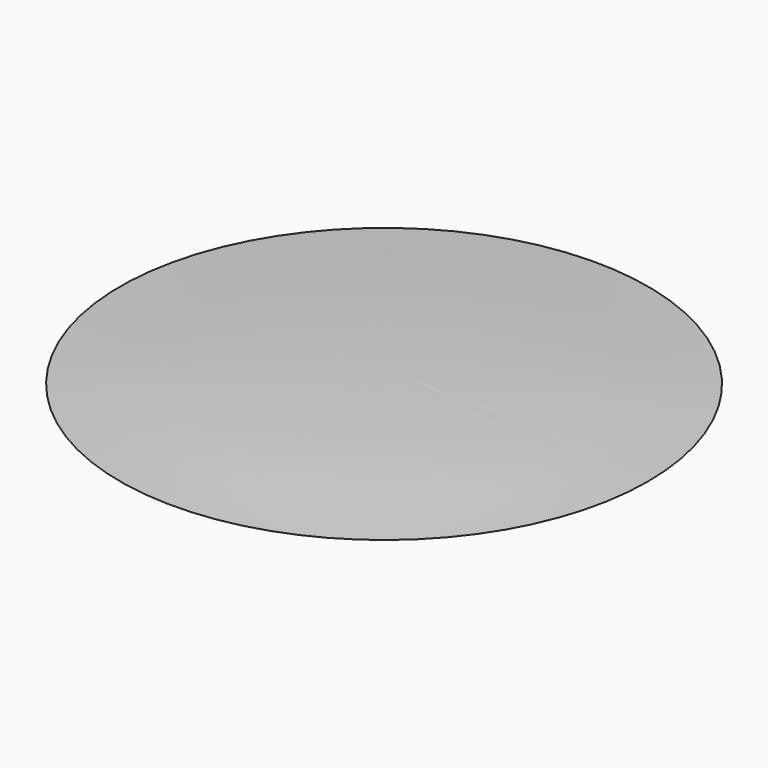
from build123d import *


# Not quite as in the source:
# - the program builds the solid bodies; features that only make, move or delete a surface that nothing else refers to are left out


with BuildPart() as f2:
    # F1 (on Front) → F2 (revolve)
    with BuildSketch(Plane.XZ):
        with BuildLine():
            add(Edge.make_bspline(
                [(1778, 0), (1221.7320122719, -33.1106260419), (1025.1461047695, -74.3691073626), (0, -74.3691073626)],
                knots=[0, 0, 0, 0, 1779.5546533136, 1779.5546533136, 1779.5546533136, 1779.5546533136], degree=3))
            add(Edge.make_bspline(
                [(1778, 0), (1221.7320122719, 33.1106260419), (1025.1461047695, 74.3691073626), (0, 74.3691073626)],
                knots=[0, 0, 0, 0, 1779.5546533136, 1779.5546533136, 1779.5546533136, 1779.5546533136], degree=3))
            Line((0, 74.3691073626), (0, -74.3691073626))
        make_face()
    revolve(axis=Axis((0, 0, -1.8308926374), (0, 0, -1)))


solid = f2.part
